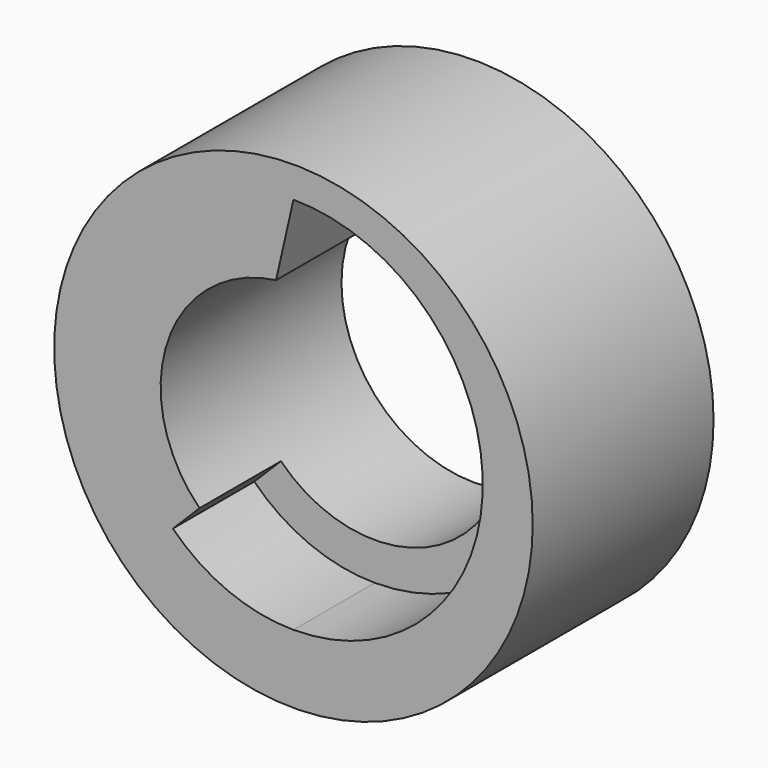
from build123d import *

# Parameters (mm, degrees)
F0_R            = 12.7
F0_R_2          = 7.05
F1_DEPTH        = 12
F3_DEPTH        = 5.4
F4_R            = 1.5
F5_DEPTH        = 2
F5_COPIES_COUNT = 10


# Not quite as in the source:
# - a pattern or mirror of a feature is missing from the dataset's text; its kind, count and spacing are read off the source's solid


with BuildPart() as f1:
    # F0 (on Front) → F1 (new body)
    with BuildSketch(Plane.XZ):
        Circle(F0_R)
        Circle(F0_R_2, mode=Mode.SUBTRACT)
    extrude(amount=F1_DEPTH)

    # F2 (on face) → F3 (cut)
    with BuildSketch(Plane.XZ.offset(12)):
        with BuildLine():
            Line((-4.9851028074, -4.9851028074), (-6.3993163697, -6.3993163697))
            ThreePointArc((-6.3993163697, -6.3993163697), (-3.4632850629, -8.3611097692), (0, -9.05))
            ThreePointArc((0, -9.05), (10.05, 1), (0, 11.05))
            Line((0, 11.05), (-0.9218489985, 6.9894702535))
            ThreePointArc((-0.9218489985, 6.9894702535), (6.6761231195, -2.2653653334), (-4.9851028074, -4.9851028074))
        make_face()
    extrude(amount=-F3_DEPTH, mode=Mode.SUBTRACT)

    # F4 (on face) → F5 (cut)
    with BuildSketch(Plane(origin=(0, 0, 0), x_dir=(-1, 0, 0), z_dir=(0, 1, 0))):
        with Locations((0, 9.875)):
            Circle(F4_R)
    f5 = extrude(amount=-F5_DEPTH, mode=Mode.SUBTRACT)

    # F5_copies: F5 ×10 about axis
    f5_copies_axis = Axis((0, 0, 0), (0, 1, 0))
    for i in range(1, F5_COPIES_COUNT):
        add(f5.rotate(f5_copies_axis, i * 360 / F5_COPIES_COUNT), mode=Mode.SUBTRACT)


solid = f1.part
